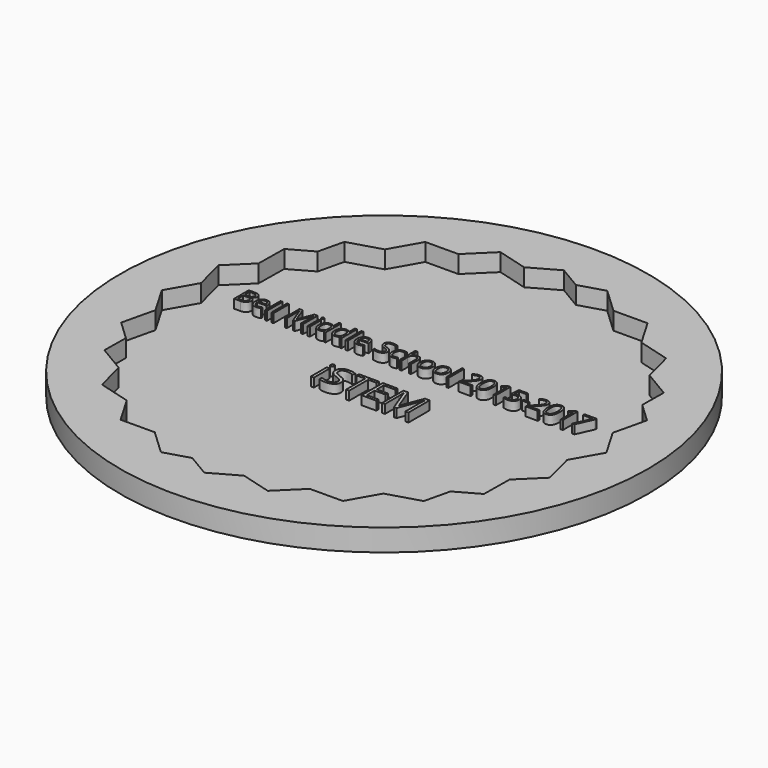
from build123d import *

# Parameters (mm, degrees)
F0_R           = 38.1
F1_DEPTH       = 3.175
F3_DEPTH       = 2.54
F4_TEXT_SIZE   = 3.7081983667
F4_TEXT_SIZE_2 = 5.3588200697
F5_DEPTH       = 1.27


# Not quite as in the source:
# - Text() gives the source's letters only with a copy of the font that has no kerning and outlines rounded to 1/6400 em; it was checked with that copy


with BuildPart() as f1:
    # F0 (on Top) → F1 (new body)
    with BuildSketch(Plane.XY):
        Circle(F0_R)
    extrude(amount=F1_DEPTH)

    # F2 (on face) → F3 (cut)
    with BuildSketch(Plane.XY.offset(3.175)):
        Polygon((-16.7539807155, -22.2307116947), (-20.2813434379, -20.1346489786), (-18.2313309667, -23.6422477825), (-14.0041852642, -24.8207506786), align=None)
        Polygon((-15.8280923204, -27.7542213045), (-10.9174468457, -27.7281570579), (-14.0041852642, -24.8207506786), (-18.2313309667, -23.6422477825), align=None)
        Polygon((-7.5328270782, -27.7101925021), (-3.7128362491, -27.6899171262), (-10.9733600143, -25.6657265999), align=None)
        Polygon((0.2854385279, -28.8046121795), (-3.7128362491, -27.6899171262), (-7.5328270782, -27.7101925021), (-3.6848346955, -29.9967827964), align=None)
        Polygon((3.5707460553, -29.7205362351), (7.2964457928, -27.6314831294), (4.1364409877, -27.6482554956), (0.2854385279, -28.8046121795), align=None)
        Polygon((11.3591216989, -27.6099196532), (7.2964457928, -27.6314831294), (3.5707460553, -29.7205362351), (7.9575307916, -30.9435455373), align=None)
        Polygon((14.4933079966, -24.5383555374), (10.875370714, -25.6247287615), (7.2964457928, -27.6314831294), (11.3591216989, -27.6099196532), align=None)
        Polygon((16.1218145518, -27.5846406951), (18.5545649894, -23.3188648418), (14.4933079966, -24.5383555374), (11.3591216989, -27.6099196532), align=None)
        Polygon((21.8758711357, 17.4063907244), (20.2813434379, 20.1346489786), (16.7539807155, 22.2307116947), align=None)
        Polygon((20.2313171115, -20.3787158631), (22.1237535355, -17.0603690749), (16.7404912349, -22.3360718372), align=None)
        Polygon((25.0882451575, -14.1551090734), (22.1237535355, -17.0603690749), (20.2313171115, -20.3787158631), (24.1355585858, -18.1895518532), align=None)
        Polygon((27.5241124213, -11.7679113232), (27.5777892307, -7.4968341508), (26.0123121234, -10.2418647712), (25.0882451575, -14.1551090734), align=None)
        Polygon((29.5904526656, -3.9676718707), (27.5777892307, -7.4968341508), (27.5241124213, -11.7679113232), (30.7766619143, -8.5803489518), align=None)
        Polygon((28.4974932607, 0.2823951412), (27.6293514295, -3.3940170668), (27.5777892307, -7.4968341508), (29.5904526656, -3.9676718707), align=None)
        Polygon((31.9499068721, 0.1695806094), (29.4720118351, 4.4092922161), (28.4974932607, 0.2823951412), (29.5904526656, -3.9676718707), align=None)
        Polygon((27.7641441897, 7.331476639), (25.8365897845, 10.6295480513), (27.7138512493, 3.3296547627), align=None)
        Polygon((24.8028066296, 14.6495031061), (25.8365897845, 10.6295480513), (27.7641441897, 7.331476639), (27.8203932812, 11.8072309432), align=None)
        Polygon((23.953366366, 17.9526249119), (20.2813434379, 20.1346489786), (21.8758711357, 17.4063907244), (24.8028066296, 14.6495031061), align=None)
        Polygon((22.8191311227, 22.3631965856), (18.2313309667, 23.6422477825), (20.2813434379, 20.1346489786), (23.953366366, 17.9526249119), align=None)
        Polygon((20.2813434379, 20.1346489786), (18.2313309667, 23.6422477825), (14.0041852642, 24.8207506786), (16.7539807155, 22.2307116947), align=None)
        Polygon((18.2313309667, 23.6422477825), (15.8280923204, 27.7542213045), (10.9174468457, 27.7281570579), (14.0041852642, 24.8207506786), align=None)
        Polygon((3.7128362491, 27.6899171262), (7.5328270782, 27.7101925021), (3.6848346955, 29.9967827964), (-0.2854385279, 28.8046121795), align=None)
        Polygon((-7.2964457928, 27.6314831294), (-4.1364409877, 27.6482554956), (-0.2854385279, 28.8046121795), (-3.5707460553, 29.7205362351), align=None)
        Polygon((10.9733600143, 25.6657265999), (7.5328270782, 27.7101925021), (3.7128362491, 27.6899171262), align=None)
        Polygon((-10.875370714, 25.6247287615), (-7.2964457928, 27.6314831294), (-11.3591216989, 27.6099196532), (-14.4933079966, 24.5383555374), align=None)
        Polygon((-11.3591216989, 27.6099196532), (-7.2964457928, 27.6314831294), (-3.5707460553, 29.7205362351), (-7.9575307916, 30.9435455373), align=None)
        Polygon((-14.4933079966, 24.5383555374), (-11.3591216989, 27.6099196532), (-16.1218145518, 27.5846406951), (-18.5545649894, 23.3188648418), align=None)
        Polygon((-22.1237535355, 17.0603690749), (-16.7404912349, 22.3360718372), (-20.2313171115, 20.3787158631), align=None)
        Polygon((-22.1237535355, 17.0603690749), (-20.2313171115, 20.3787158631), (-24.1355585858, 18.1895518532), (-25.0882451575, 14.1551090734), align=None)
        Polygon((-27.5777892307, 7.4968341508), (-26.0123121234, 10.2418647712), (-25.0882451575, 14.1551090734), (-27.5241124213, 11.7679113232), align=None)
        Polygon((-29.5904526656, 3.9676718707), (-27.5777892307, 7.4968341508), (-27.5241124213, 11.7679113232), (-30.7766619143, 8.5803489518), align=None)
        Polygon((-27.6293514295, 3.3940170668), (-27.5777892307, 7.4968341508), (-29.5904526656, 3.9676718707), (-28.4974932607, -0.2823951412), align=None)
        Polygon((-28.4974932607, -0.2823951412), (-29.5904526656, 3.9676718707), (-31.9499068721, -0.1695806094), (-29.4720118351, -4.4092922161), align=None)
        Polygon((-25.8365897845, -10.6295480513), (-27.7138512493, -3.3296547627), (-27.7641441897, -7.331476639), align=None)
        Polygon((-20.2813434379, -20.1346489786), (-21.8758711357, -17.4063907244), (-24.8028066296, -14.6495031061), (-23.953366366, -17.9526249119), align=None)
        Polygon((-25.8365897845, -10.6295480513), (-27.7641441897, -7.331476639), (-27.8203932812, -11.8072309432), (-24.8028066296, -14.6495031061), align=None)
        Polygon((-24.8028066296, -14.6495031061), (-27.8203932812, -11.8072309432), (-27.8683882635, -15.6262037078), (-23.953366366, -17.9526249119), align=None)
        Polygon((-27.8203932812, -11.8072309432), (-27.7641441897, -7.331476639), (-29.4720118351, -4.4092922161), (-30.6005813396, -9.1885650892), align=None)
        Polygon((-27.7641441897, -7.331476639), (-27.7138512493, -3.3296547627), (-28.4974932607, -0.2823951412), (-29.4720118351, -4.4092922161), align=None)
        Polygon((-27.7138512493, -3.3296547627), (-27.6293514295, 3.3940170668), (-28.4974932607, -0.2823951412), align=None)
        Polygon((-27.6293514295, 3.3940170668), (-26.0123121234, 10.2418647712), (-27.5777892307, 7.4968341508), align=None)
        Polygon((-26.0123121234, 10.2418647712), (-22.1237535355, 17.0603690749), (-25.0882451575, 14.1551090734), align=None)
        Polygon((-25.0882451575, 14.1551090734), (-24.1355585858, 18.1895518532), (-27.4668835074, 16.3216303448), (-27.5241124213, 11.7679113232), align=None)
        Polygon((-24.1355585858, 18.1895518532), (-20.2313171115, 20.3787158631), (-18.5545649894, 23.3188648418), (-23.2578214614, 21.9065982661), align=None)
        Polygon((7.5328270782, 27.7101925021), (10.9174468457, 27.7281570579), (7.3427598783, 31.0951633553), (3.6848346955, 29.9967827964), align=None)
        Polygon((-0.2854385279, 28.8046121795), (3.6848346955, 29.9967827964), (0.4015047561, 31.9478340526), (-3.5707460553, 29.7205362351), align=None)
        Polygon((-4.1364409877, 27.6482554956), (3.7128362491, 27.6899171262), (-0.2854385279, 28.8046121795), align=None)
        Polygon((-10.875370714, 25.6247287615), (-4.1364409877, 27.6482554956), (-7.2964457928, 27.6314831294), align=None)
        Polygon((-20.2313171115, 20.3787158631), (-16.7404912349, 22.3360718372), (-14.4933079966, 24.5383555374), (-18.5545649894, 23.3188648418), align=None)
        Polygon((27.8203932812, 11.8072309432), (27.7641441897, 7.331476639), (29.4720118351, 4.4092922161), (30.6005813396, 9.1885650892), align=None)
        Polygon((27.8683882635, 15.6262037078), (23.953366366, 17.9526249119), (24.8028066296, 14.6495031061), (27.8203932812, 11.8072309432), align=None)
        Polygon((29.4720118351, 4.4092922161), (27.7641441897, 7.331476639), (27.7138512493, 3.3296547627), (28.4974932607, 0.2823951412), align=None)
        Polygon((27.4668835074, -16.3216303448), (27.5241124213, -11.7679113232), (25.0882451575, -14.1551090734), (24.1355585858, -18.1895518532), align=None)
        Polygon((24.1355585858, -18.1895518532), (20.2313171115, -20.3787158631), (18.5545649894, -23.3188648418), (23.2578214614, -21.9065982661), align=None)
        Polygon((18.5545649894, -23.3188648418), (20.2313171115, -20.3787158631), (16.7404912349, -22.3360718372), (14.4933079966, -24.5383555374), align=None)
        Polygon((-0.4015047561, -31.9478340526), (3.5707460553, -29.7205362351), (0.2854385279, -28.8046121795), (-3.6848346955, -29.9967827964), align=None)
        Polygon((-3.6848346955, -29.9967827964), (-7.5328270782, -27.7101925021), (-10.9174468457, -27.7281570579), (-7.3427598783, -31.0951633553), align=None)
        Polygon((-10.9174468457, -27.7281570579), (-7.5328270782, -27.7101925021), (-10.9733600143, -25.6657265999), (-14.0041852642, -24.8207506786), align=None)
        Polygon((14.0041852642, 24.8207506786), (10.9174468457, 27.7281570579), (7.5328270782, 27.7101925021), (10.9733600143, 25.6657265999), align=None)
        Polygon((25.8365897845, 10.6295480513), (21.8758711357, 17.4063907244), (16.7539807155, 22.2307116947), (10.9733600143, 25.6657265999), (3.7128362491, 27.6899171262), (-4.1364409877, 27.6482554956), (-10.875370714, 25.6247287615), (-16.7404912349, 22.3360718372), (-22.1237535355, 17.0603690749), (-26.0123121234, 10.2418647712), (-27.6293514295, 3.3940170668), (-27.7138512493, -3.3296547627), (-25.8365897845, -10.6295480513), (-21.8758711357, -17.4063907244), (-16.7539807155, -22.2307116947), (-10.9733600143, -25.6657265999), (-3.7128362491, -27.6899171262), (4.1364409877, -27.6482554956), (10.875370714, -25.6247287615), (16.7404912349, -22.3360718372), (22.1237535355, -17.0603690749), (26.0123121234, -10.2418647712), (27.6293514295, -3.3940170668), (27.7138512493, 3.3296547627), align=None)
        Polygon((27.5777892307, -7.4968341508), (27.6293514295, -3.3940170668), (26.0123121234, -10.2418647712), align=None)
        Polygon((25.0882451575, -14.1551090734), (26.0123121234, -10.2418647712), (22.1237535355, -17.0603690749), align=None)
        Polygon((7.2964457928, -27.6314831294), (10.875370714, -25.6247287615), (4.1364409877, -27.6482554956), align=None)
        Polygon((14.4933079966, -24.5383555374), (16.7404912349, -22.3360718372), (10.875370714, -25.6247287615), align=None)
        Polygon((0.2854385279, -28.8046121795), (4.1364409877, -27.6482554956), (-3.7128362491, -27.6899171262), align=None)
        Polygon((-14.0041852642, -24.8207506786), (-10.9733600143, -25.6657265999), (-16.7539807155, -22.2307116947), align=None)
        Polygon((-18.2313309667, -23.6422477825), (-20.2813434379, -20.1346489786), (-23.953366366, -17.9526249119), (-22.8191311227, -22.3631965856), align=None)
        Polygon((-21.8758711357, -17.4063907244), (-25.8365897845, -10.6295480513), (-24.8028066296, -14.6495031061), align=None)
        Polygon((-16.7539807155, -22.2307116947), (-21.8758711357, -17.4063907244), (-20.2813434379, -20.1346489786), align=None)
        Polygon((16.7539807155, 22.2307116947), (14.0041852642, 24.8207506786), (10.9733600143, 25.6657265999), align=None)
        Polygon((-16.7404912349, 22.3360718372), (-10.875370714, 25.6247287615), (-14.4933079966, 24.5383555374), align=None)
        Polygon((24.8028066296, 14.6495031061), (21.8758711357, 17.4063907244), (25.8365897845, 10.6295480513), align=None)
        Polygon((28.4974932607, 0.2823951412), (27.7138512493, 3.3296547627), (27.6293514295, -3.3940170668), align=None)
    extrude(amount=-F3_DEPTH, mode=Mode.SUBTRACT)

    # F4 (on face) → F5 (join)
    with BuildSketch(Plane.XY.offset(0.635)):
        with Locations((-26.1798842968, 5.2130704084)):
            Text('Bell Middle School 2015-2017', F4_TEXT_SIZE, font='Open Sans', text_align=(TextAlign.LEFT, TextAlign.BOTTOM))
        with Locations((-7.665932033, -4.2137248383)):
            Text('iSTEM', F4_TEXT_SIZE_2, font='Open Sans', text_align=(TextAlign.LEFT, TextAlign.BOTTOM))
    extrude(amount=F5_DEPTH)


solid = f1.part
